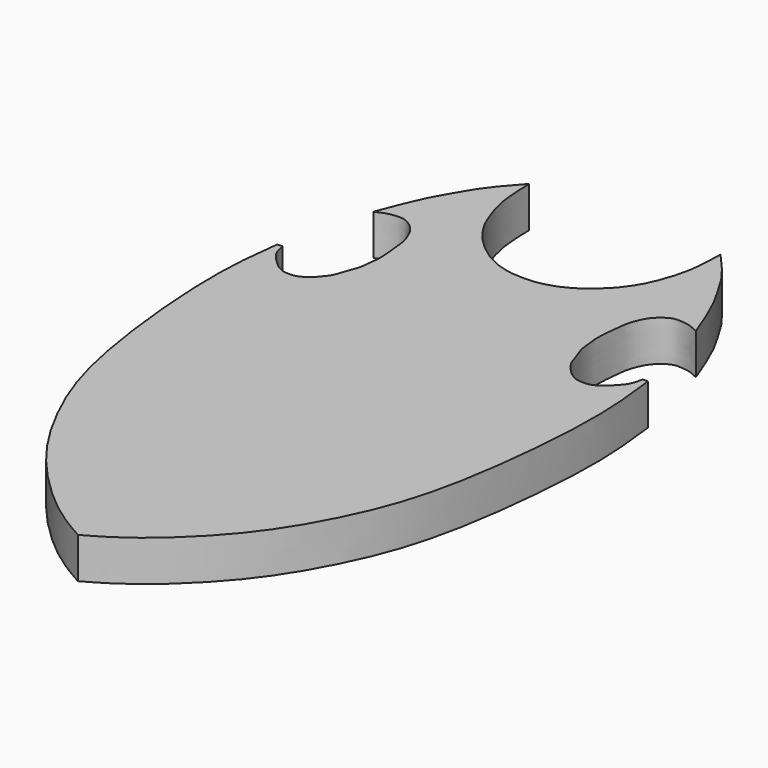
from build123d import *

# Parameters (mm, degrees)
F1_DEPTH = 5


with BuildPart() as f1:
    # F0 (on Top) → F1 (new body)
    with BuildSketch(Plane.XY):
        with BuildLine():
            add(Edge.make_bspline(
                [(-57.5626678765, 42.6406040788), (-57.9080562921, 39.8362415044), (-58.7477625906, 33.018291596), (-56.7466207027, 13.2638324141), (-52.8291963564, 2.9733901681), (-47.5742402511, -6.1031265313), (-39.8588097864, -13.4804555699), (-36.3235197152, -15.4765553984), (-34.8331145942, -16.3180697709)],
                knots=[0, 0, 0, 0, 0.1571384934, 0.3820341872, 0.5524442159, 0.7154761313, 0.880050626, 1, 1, 1, 1], degree=3))
            Line((-34.8331145942, -16.3180697709), (-34.8331145942, 51.9118197262))
            add(Edge.make_bspline(
                [(-34.8331145942, 51.9118197262), (-35.2119563545, 51.9185959347), (-35.9580977588, 51.9319419017), (-37.0348440475, 52.1008517041), (-37.751583743, 52.3413787982), (-38.5534512152, 52.5661302145), (-39.1045545857, 52.8892692232), (-39.9530807974, 53.242750596), (-40.6024267483, 53.772012849), (-41.4634310205, 54.3811984195), (-42.0706109603, 54.9524802776), (-42.9037456065, 55.720108633), (-43.4259718244, 56.3914555617), (-43.9234358745, 57.0589950526), (-44.2302322209, 57.5786939094), (-44.7376887484, 58.3206849113), (-45.4837434911, 60.2315423487), (-45.9027412703, 61.4635918917), (-46.1149072684, 62.587386495), (-46.2910492058, 63.1994502703), (-46.3665046988, 64.0072029965), (-46.457462946, 64.8854328545), (-46.519316114, 65.8331058884), (-46.5460145844, 66.9017915796), (-46.5613380075, 67.5151571631)],
                knots=[0, 0, 0, 0, 0.0493610993, 0.0972183213, 0.1377301504, 0.1791101827, 0.2163531524, 0.2599263059, 0.3028340171, 0.3496999184, 0.3925564746, 0.4412704382, 0.4846073731, 0.5261866583, 0.5613175523, 0.6048162611, 0.6709705647, 0.7254358561, 0.7735910677, 0.8104237672, 0.8515345399, 0.8947116941, 0.939570424, 1, 1, 1, 1], degree=3))
            add(Edge.make_bspline(
                [(-46.5613380075, 67.5151571631), (-47.2280532122, 66.7531962196), (-47.8947684169, 65.9912352761), (-48.5614836216, 65.2292743325)],
                knots=[0, 0, 0, 0, 3.0374072485, 3.0374072485, 3.0374072485, 3.0374072485], degree=3))
            add(Edge.make_bspline(
                [(-48.5614836216, 65.2292743325), (-48.9735694738, 64.7136433972), (-49.7863729956, 63.6966043776), (-50.6916211477, 62.0419000493), (-51.5394060192, 60.7181023455), (-52.3324629663, 59.2186716244), (-52.9254322483, 57.9124520433), (-53.7256402788, 56.0234412783), (-54.3032039704, 54.4922006053), (-54.6109952031, 53.6815354107)],
                knots=[0, 0, 0, 0, 0.1473527895, 0.2906803309, 0.4229073329, 0.5579037502, 0.6834554494, 0.8324703555, 1, 1, 1, 1], degree=3))
            add(Edge.make_bspline(
                [(-54.6109952031, 53.6815354107), (-54.1490167087, 53.8989858417), (-53.3838791321, 54.2576504993), (-52.2461372119, 54.37354881), (-51.3518225299, 54.3873217778), (-50.5313887829, 53.9583071647), (-49.5211267731, 53.1279307693), (-48.8411316868, 51.797376606), (-48.4783197566, 50.6331243975), (-48.4119479233, 49.8877598597), (-48.3026124514, 48.9386253318), (-48.1973480176, 48.009616531), (-48.071268063, 46.2101292746), (-48.3446637999, 44.8877932345), (-48.333153973, 43.9230372084), (-49.1109571235, 42.0884729348), (-49.3749084991, 41.0183008159), (-50.0069662335, 40.2196283926), (-50.7492629002, 39.336743191), (-51.5427317075, 38.8453486879), (-52.1317926314, 38.5710112066), (-53.4087673752, 38.5344057135), (-53.9588643746, 38.7602882902), (-54.4148685339, 38.9915837878), (-54.6061547794, 39.1268395676)],
                knots=[0, 0, 0, 0, 0.0445420475, 0.0845400391, 0.1197214949, 0.1554017993, 0.1984744889, 0.2451509962, 0.2866397794, 0.3193912307, 0.3554993097, 0.3927526907, 0.4436884008, 0.4874368635, 0.5247166115, 0.5776970761, 0.6179417164, 0.6554167928, 0.6964030165, 0.732305622, 0.7631963792, 0.8049886746, 0.8359919351, 0.8636682784, 0.8636682784, 0.8636682784, 0.8636682784], degree=3))
            add(Edge.make_bspline(
                [(-54.6061547794, 39.1268395676), (-54.6592591816, 39.1643889341), (-54.7889448477, 39.2644677015), (-54.8995408977, 39.3780040162), (-54.9651332554, 39.4462250728)],
                knots=[0.8636682784, 0.8636682784, 0.8636682784, 0.8636682784, 0.8713517146, 0.8831028995, 0.8831028995, 0.8831028995, 0.8831028995], degree=3))
            add(Edge.make_bspline(
                [(-54.9651332554, 39.4462250728), (-55.0422718783, 39.5157558174), (-55.1496780772, 39.6135140467), (-55.2724769461, 39.7270938328), (-55.3011469605, 39.7537806896)],
                knots=[0.1606199003, 0.1606199003, 0.1606199003, 0.1606199003, 0.2554193728, 0.2834344333, 0.2834344333, 0.2834344333, 0.2834344333], degree=3))
            add(Edge.make_bspline(
                [(-55.3011469605, 39.7537806896), (-55.3239737809, 39.7694364315), (-55.5998529876, 39.9433833713), (-56.0474560794, 39.9919072855), (-56.1453497064, 40.5782185414), (-56.1541033084, 40.6599148874)],
                knots=[0.9022974714, 0.9022974714, 0.9022974714, 0.9022974714, 0.905798506, 0.9433289244, 0.9488544637, 0.9488544637, 0.9488544637, 0.9488544637], degree=3))
            add(Edge.make_bspline(
                [(-56.1541033084, 40.6599148874), (-56.2472964392, 40.7810745041), (-56.6797268519, 41.4080624482), (-56.8130311576, 42.0925613255), (-56.9197610021, 42.6406040788)],
                knots=[0.5429117903, 0.5429117903, 0.5429117903, 0.5429117903, 0.6340331748, 1, 1, 1, 1], degree=3))
            add(Edge.make_bspline(
                [(-56.9197610021, 42.6406040788), (-57.1340632935, 42.6406040788), (-57.348365585, 42.6406040788), (-57.5626678765, 42.6406040788)],
                knots=[0, 0, 0, 0, 0.6429068744, 0.6429068744, 0.6429068744, 0.6429068744], degree=3))
        make_face()
        with BuildLine():
            Line((-34.8331145942, 51.9118197262), (-34.8331145942, -16.3180697709))
            add(Edge.make_bspline(
                [(-12.103561312, 42.6406040788), (-11.7581728963, 39.8362415044), (-10.9184665978, 33.018291596), (-12.9196084857, 13.2638324141), (-16.8370328321, 2.9733901681), (-22.0919889373, -6.1031265313), (-29.8074194021, -13.4804555699), (-33.3427094733, -15.4765553984), (-34.8331145942, -16.3180697709)],
                knots=[0, 0, 0, 0, 0.1571384934, 0.3820341872, 0.5524442159, 0.7154761313, 0.880050626, 1, 1, 1, 1], degree=3))
            add(Edge.make_bspline(
                [(-12.7464681864, 42.6406040788), (-12.5321658949, 42.6406040788), (-12.3178636034, 42.6406040788), (-12.103561312, 42.6406040788)],
                knots=[0, 0, 0, 0, 0.6429068744, 0.6429068744, 0.6429068744, 0.6429068744], degree=3))
            add(Edge.make_bspline(
                [(-13.51212588, 40.6599148874), (-13.4189327492, 40.7810745041), (-12.9865023366, 41.4080624482), (-12.8531980309, 42.0925613255), (-12.7464681864, 42.6406040788)],
                knots=[0.5429117903, 0.5429117903, 0.5429117903, 0.5429117903, 0.6340331748, 1, 1, 1, 1], degree=3))
            add(Edge.make_bspline(
                [(-14.3650822279, 39.7537806896), (-14.3422554076, 39.7694364315), (-14.0663762008, 39.9433833713), (-13.618773109, 39.9919072855), (-13.5208794821, 40.5782185414), (-13.51212588, 40.6599148874)],
                knots=[0.9022974714, 0.9022974714, 0.9022974714, 0.9022974714, 0.905798506, 0.9433289244, 0.9488544637, 0.9488544637, 0.9488544637, 0.9488544637], degree=3))
            add(Edge.make_bspline(
                [(-14.7010959331, 39.4462250728), (-14.6239573101, 39.5157558174), (-14.5165511113, 39.6135140467), (-14.3937522423, 39.7270938328), (-14.3650822279, 39.7537806896)],
                knots=[0.1606199003, 0.1606199003, 0.1606199003, 0.1606199003, 0.2554193728, 0.2834344333, 0.2834344333, 0.2834344333, 0.2834344333], degree=3))
            add(Edge.make_bspline(
                [(-15.0600744091, 39.1268395676), (-15.0069700068, 39.1643889341), (-14.8772843408, 39.2644677015), (-14.7666882907, 39.3780040162), (-14.7010959331, 39.4462250728)],
                knots=[0.8636682784, 0.8636682784, 0.8636682784, 0.8636682784, 0.8713517146, 0.8831028995, 0.8831028995, 0.8831028995, 0.8831028995], degree=3))
            add(Edge.make_bspline(
                [(-15.0552339853, 53.6815354107), (-15.5172124798, 53.8989858417), (-16.2823500564, 54.2576504993), (-17.4200919766, 54.37354881), (-18.3144066585, 54.3873217778), (-19.1348404055, 53.9583071647), (-20.1451024154, 53.1279307693), (-20.8250975017, 51.797376606), (-21.1879094318, 50.6331243975), (-21.2542812651, 49.8877598597), (-21.363616737, 48.9386253318), (-21.4688811708, 48.009616531), (-21.5949611255, 46.2101292746), (-21.3215653885, 44.8877932345), (-21.3330752154, 43.9230372084), (-20.555272065, 42.0884729348), (-20.2913206893, 41.0183008159), (-19.6592629549, 40.2196283926), (-18.9169662882, 39.336743191), (-18.123497481, 38.8453486879), (-17.5344365571, 38.5710112066), (-16.2574618133, 38.5344057135), (-15.7073648139, 38.7602882902), (-15.2513606546, 38.9915837878), (-15.0600744091, 39.1268395676)],
                knots=[0, 0, 0, 0, 0.0445420475, 0.0845400391, 0.1197214949, 0.1554017993, 0.1984744889, 0.2451509962, 0.2866397794, 0.3193912307, 0.3554993097, 0.3927526907, 0.4436884008, 0.4874368635, 0.5247166115, 0.5776970761, 0.6179417164, 0.6554167928, 0.6964030165, 0.732305622, 0.7631963792, 0.8049886746, 0.8359919351, 0.8636682784, 0.8636682784, 0.8636682784, 0.8636682784], degree=3))
            add(Edge.make_bspline(
                [(-21.1047455668, 65.2292743325), (-20.6926597146, 64.7136433972), (-19.8798561928, 63.6966043776), (-18.9746080407, 62.0419000493), (-18.1268231693, 60.7181023455), (-17.3337662222, 59.2186716244), (-16.7407969402, 57.9124520433), (-15.9405889096, 56.0234412783), (-15.363025218, 54.4922006053), (-15.0552339853, 53.6815354107)],
                knots=[0, 0, 0, 0, 0.1473527895, 0.2906803309, 0.4229073329, 0.5579037502, 0.6834554494, 0.8324703555, 1, 1, 1, 1], degree=3))
            add(Edge.make_bspline(
                [(-23.104891181, 67.5151571631), (-22.4381759763, 66.7531962196), (-21.7714607716, 65.9912352761), (-21.1047455668, 65.2292743325)],
                knots=[0, 0, 0, 0, 3.0374072485, 3.0374072485, 3.0374072485, 3.0374072485], degree=3))
            add(Edge.make_bspline(
                [(-34.8331145942, 51.9118197262), (-34.4542728339, 51.9185959347), (-33.7081314296, 51.9319419017), (-32.6313851409, 52.1008517041), (-31.9146454455, 52.3413787982), (-31.1127779733, 52.5661302145), (-30.5616746027, 52.8892692232), (-29.713148391, 53.242750596), (-29.0638024401, 53.772012849), (-28.202798168, 54.3811984195), (-27.5956182281, 54.9524802776), (-26.762483582, 55.720108633), (-26.240257364, 56.3914555617), (-25.7427933139, 57.0589950526), (-25.4359969675, 57.5786939094), (-24.92854044, 58.3206849113), (-24.1824856973, 60.2315423487), (-23.7634879182, 61.4635918917), (-23.55132192, 62.587386495), (-23.3751799827, 63.1994502703), (-23.2997244896, 64.0072029965), (-23.2087662424, 64.8854328545), (-23.1469130745, 65.8331058884), (-23.120214604, 66.9017915796), (-23.104891181, 67.5151571631)],
                knots=[0, 0, 0, 0, 0.0493610993, 0.0972183213, 0.1377301504, 0.1791101827, 0.2163531524, 0.2599263059, 0.3028340171, 0.3496999184, 0.3925564746, 0.4412704382, 0.4846073731, 0.5261866583, 0.5613175523, 0.6048162611, 0.6709705647, 0.7254358561, 0.7735910677, 0.8104237672, 0.8515345399, 0.8947116941, 0.939570424, 1, 1, 1, 1], degree=3))
        make_face()
        with BuildLine():
            add(Edge.make_bspline(
                [(-55.3011469605, 39.7537806896), (-55.566690544, 40.0009561348), (-55.8887264446, 40.3149006271), (-56.1541033084, 40.6599148874)],
                knots=[0.2834344333, 0.2834344333, 0.2834344333, 0.2834344333, 0.5429117903, 0.5429117903, 0.5429117903, 0.5429117903], degree=3))
            add(Edge.make_bspline(
                [(-55.3011469605, 39.7537806896), (-55.3239737809, 39.7694364315), (-55.5998529876, 39.9433833713), (-56.0474560794, 39.9919072855), (-56.1453497064, 40.5782185414), (-56.1541033084, 40.6599148874)],
                knots=[0.9022974714, 0.9022974714, 0.9022974714, 0.9022974714, 0.905798506, 0.9433289244, 0.9488544637, 0.9488544637, 0.9488544637, 0.9488544637], degree=3))
        make_face()
        with BuildLine():
            add(Edge.make_bspline(
                [(-14.3650822279, 39.7537806896), (-14.3422554076, 39.7694364315), (-14.0663762008, 39.9433833713), (-13.618773109, 39.9919072855), (-13.5208794821, 40.5782185414), (-13.51212588, 40.6599148874)],
                knots=[0.9022974714, 0.9022974714, 0.9022974714, 0.9022974714, 0.905798506, 0.9433289244, 0.9488544637, 0.9488544637, 0.9488544637, 0.9488544637], degree=3))
            add(Edge.make_bspline(
                [(-14.3650822279, 39.7537806896), (-14.0995386444, 40.0009561348), (-13.7775027438, 40.3149006271), (-13.51212588, 40.6599148874)],
                knots=[0.2834344333, 0.2834344333, 0.2834344333, 0.2834344333, 0.5429117903, 0.5429117903, 0.5429117903, 0.5429117903], degree=3))
        make_face()
        with BuildLine():
            add(Edge.make_bspline(
                [(-54.6061547794, 39.1268395676), (-54.6592591816, 39.1643889341), (-54.7889448477, 39.2644677015), (-54.8995408977, 39.3780040162), (-54.9651332554, 39.4462250728)],
                knots=[0.8636682784, 0.8636682784, 0.8636682784, 0.8636682784, 0.8713517146, 0.8831028995, 0.8831028995, 0.8831028995, 0.8831028995], degree=3))
            add(Edge.make_bspline(
                [(-54.6061547794, 39.1268395676), (-54.7202955635, 39.2276289267), (-54.8344363476, 39.3284182859), (-54.9651332554, 39.4462250728)],
                knots=[0, 0, 0, 0, 0.1606199003, 0.1606199003, 0.1606199003, 0.1606199003], degree=3))
        make_face()
        with BuildLine():
            add(Edge.make_bspline(
                [(-15.0600744091, 39.1268395676), (-14.945933625, 39.2276289267), (-14.8317928408, 39.3284182859), (-14.7010959331, 39.4462250728)],
                knots=[0, 0, 0, 0, 0.1606199003, 0.1606199003, 0.1606199003, 0.1606199003], degree=3))
            add(Edge.make_bspline(
                [(-15.0600744091, 39.1268395676), (-15.0069700068, 39.1643889341), (-14.8772843408, 39.2644677015), (-14.7666882907, 39.3780040162), (-14.7010959331, 39.4462250728)],
                knots=[0.8636682784, 0.8636682784, 0.8636682784, 0.8636682784, 0.8713517146, 0.8831028995, 0.8831028995, 0.8831028995, 0.8831028995], degree=3))
        make_face()
    extrude(amount=F1_DEPTH)


solid = f1.part
